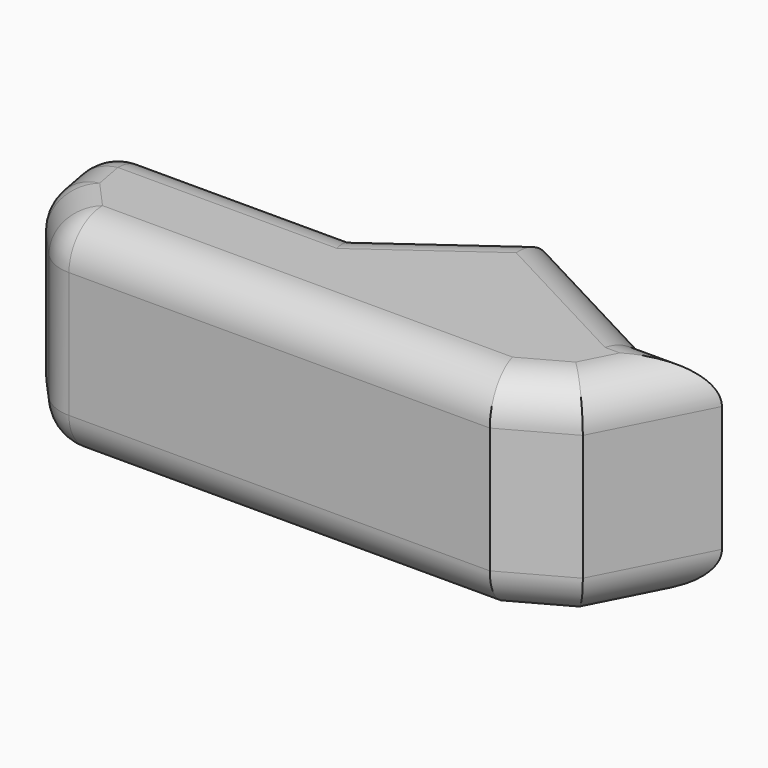
from build123d import *

# Parameters (mm, degrees)
F2_DEPTH     = 25.4
F3_R         = 5.08
F4_T1_DEPTH  = 63.7089962256
F4_T3_DEPTH  = 34.3299805756
F4_T5_DEPTH  = 39.8420593032
F4_T7_DEPTH  = 15.24
F4_T12_DEPTH = 5.08
F4_T18_DEPTH = 5.08
F4_T24_DEPTH = 5.08
F4_T30_DEPTH = 5.08
F4_T36_DEPTH = 37.6403571065
F4_T41_DEPTH = 43.8944483223
F4_T46_DEPTH = 48.4484626095
F4_T51_DEPTH = 34.2442917913
F4_T57_DEPTH = 43.8944483223
F4_T61_DEPTH = 37.6403571065
F4_T68_DEPTH = 48.4484626095
F4_T72_DEPTH = 34.2442917913


# Not quite as in the source:
# - a fillet or chamfer that OpenCascade refuses, or shapes differently, is made with other operations: its cross-section is extruded or revolved along the edge and cut away or added


with BuildPart() as f2:
    # F1 (on face) → F2 (new body)
    with BuildSketch(Plane.XY):
        Polygon((8.4329312667, 10.7982652262), (-6.5817977302, 0), (-37.6396663487, 0), (-35.5828553438, -11.0039459541), (-30.0294607878, -17.1743836254), (23.241976276, -17.1743836254), (31.0578662902, -12.8550762311), (37.6396663487, 0), (28.7953745574, 0), align=None)
    extrude(amount=F2_DEPTH)

    # F3
    f3_edges = [f2.edges().sort_by_distance(p)[0] for p in [
        (-22.110732, 0, 25.4),
        (18.614153, 5.399133, 25.4),
        (33.21752, 0, 25.4),
        (34.348766, -6.427538, 25.4),
        (27.149921, -15.01473, 25.4),
        (-3.393742, -17.174384, 25.4),
        (-32.806158, -14.089165, 25.4),
        (-36.611261, -5.501973, 25.4),
        (-32.806158, -14.089165, 0),
        (-36.611261, -5.501973, 0),
        (-35.582855, -11.003946, 12.7),
        (0.925567, 5.399133, 25.4),
    ]]
    fillet(f3_edges, radius=F3_R)

    # F4: fillet of radius 5.08 on 11 edges, made by hand

    # F4_s2 → F4_t1 (cut)
    with BuildSketch(Plane.YZ.offset(-27.7670199495)):
        with BuildLine():
            ThreePointArc((-12.0943836254, 0), (-15.6864860738, 1.4878975516), (-17.1743836254, 5.08))
            Line((-17.1743836254, 5.08), (-17.1743836254, 0))
            Line((-17.1743836254, 0), (-12.0943836254, 0))
        make_face()
    extrude(amount=F4_T1_DEPTH, mode=Mode.SUBTRACT)

    # F4_s4 → F4_t3 (cut)
    with BuildSketch(Plane(origin=(-0.5817443509, -0.3214902809, 0), x_dir=(0, 0, 1), z_dir=(0.8752415471, 0.4836860907, 0))):
        with BuildLine():
            ThreePointArc((0, 21.1935547384), (1.4878975516, 24.7856571868), (5.08, 26.2735547384))
            Line((5.08, 26.2735547384), (0, 26.2735547384))
            Line((0, 26.2735547384), (0, 21.1935547384))
        make_face()
    extrude(amount=F4_T3_DEPTH, mode=Mode.SUBTRACT)

    # F4_s6 → F4_t5 (cut)
    with BuildSketch(Plane(origin=(-4.5520149502, -8.8906528107, 0), x_dir=(0, 0, 1), z_dir=(0.4557383348, 0.8901137962, 0))):
        with BuildLine():
            ThreePointArc((0, 28.4235863007), (1.4878975516, 32.0156887492), (5.08, 33.5035863007))
            Line((5.08, 33.5035863007), (0, 33.5035863007))
            Line((0, 33.5035863007), (0, 28.4235863007))
        make_face()
    extrude(amount=F4_T5_DEPTH, mode=Mode.SUBTRACT)

    # F4_s8 → F4_t7 (cut)
    with BuildSketch(Plane.XY.offset(5.08)):
        with BuildLine():
            ThreePointArc((-31.5221548367, 0), (-35.430345336, -1.8346268287), (-36.5156731811, -6.0133673145))
            Line((-36.5156731811, -6.0133673145), (-37.6396663487, 0))
            Line((-37.6396663487, 0), (-31.5221548367, 0))
        make_face()
        with BuildLine():
            ThreePointArc((-27.7670199495, -17.1743836254), (-29.8337598255, -16.7349640077), (-31.5429540141, -15.4927246824))
            Line((-31.5429540141, -15.4927246824), (-30.0294607878, -17.1743836254))
            Line((-30.0294607878, -17.1743836254), (-27.7670199495, -17.1743836254))
        make_face()
    extrude(amount=F4_T7_DEPTH, mode=Mode.SUBTRACT)


with BuildPart() as f4_tool10:
    # F4_s11 → F4_t12 (new body)
    with BuildSketch(Plane.XY.offset(20.32)):
        Polygon((-27.7670199495, -12.0943836254), (-27.7670199495, -17.1743836254), (-30.0294607878, -17.1743836254), (-31.5429540141, -15.4927246824), align=None)
    extrude(amount=F4_T12_DEPTH)

    # F4_s13 → F4_t14 (revolve, cut)
    with BuildSketch(Plane(origin=(-27.7670199495, -12.0943836254, 20.32), x_dir=(0.4068385583, 0.9135000753, 0), z_dir=(0.9135000753, -0.4068385583, 0))):
        with BuildLine():
            ThreePointArc((0, -5.08), (5.08, 0), (0, 5.08))
            Line((0, 5.08), (0, -5.08))
        make_face()
    revolve(axis=Axis((-27.7670199495, -12.0943836254, 20.32), (0, 0, 1)), mode=Mode.SUBTRACT)


with BuildPart() as f2_1:
    add(f2.part)

    # F4_t9: cut F4_tool10
    add(f4_tool10.part, mode=Mode.SUBTRACT)


with BuildPart() as f4_tool16:
    # F4_s17 → F4_t18 (new body)
    with BuildSketch(Plane.XY.offset(20.32)):
        Polygon((-31.5221548367, -5.08), (-31.5221548367, 0), (-37.6396663487, 0), (-36.5156731811, -6.0133673145), align=None)
    extrude(amount=F4_T18_DEPTH)

    # F4_s19 → F4_t20 (revolve, cut)
    with BuildSketch(Plane(origin=(-31.5221548367, -5.08, 20.32), x_dir=(0.7693288384, -0.6388529865, 0), z_dir=(-0.6388529865, -0.7693288384, 0))):
        with BuildLine():
            ThreePointArc((0, -5.08), (5.08, 0), (0, 5.08))
            Line((0, 5.08), (0, -5.08))
        make_face()
    revolve(axis=Axis((-31.5221548367, -5.08, 20.32), (0, 0, 1)), mode=Mode.SUBTRACT)


with BuildPart() as f2_2:
    add(f2_1.part)

    # F4_t15: cut F4_tool16
    add(f4_tool16.part, mode=Mode.SUBTRACT)


with BuildPart() as f4_tool22:
    # F4_s23 → F4_t24 (new body)
    with BuildSketch(Plane.XY.offset(5.08)):
        Polygon((-27.7670199495, -12.0943836254), (-27.7670199495, -17.1743836254), (-30.0294607878, -17.1743836254), (-31.5429540141, -15.4927246824), align=None)
    extrude(amount=-F4_T24_DEPTH)

    # F4_s25 → F4_t26 (revolve, cut)
    with BuildSketch(Plane(origin=(-27.7670199495, -12.0943836254, 5.08), x_dir=(0.4068385583, 0.9135000753, 0), z_dir=(-0.9135000753, 0.4068385583, 0))):
        with BuildLine():
            ThreePointArc((0, -5.08), (5.08, 0), (0, 5.08))
            Line((0, 5.08), (0, -5.08))
        make_face()
    revolve(axis=Axis((-27.7670199495, -12.0943836254, 5.08), (0, 0, -1)), mode=Mode.SUBTRACT)


with BuildPart() as f2_3:
    add(f2_2.part)

    # F4_t21: cut F4_tool22
    add(f4_tool22.part, mode=Mode.SUBTRACT)


with BuildPart() as f4_tool28:
    # F4_s29 → F4_t30 (new body)
    with BuildSketch(Plane.XY.offset(5.08)):
        Polygon((-31.5221548367, -5.08), (-31.5221548367, 0), (-37.6396663487, 0), (-36.5156731811, -6.0133673145), align=None)
    extrude(amount=-F4_T30_DEPTH)

    # F4_s31 → F4_t32 (revolve, cut)
    with BuildSketch(Plane(origin=(-31.5221548367, -5.08, 5.08), x_dir=(0.7693288384, -0.6388529865, 0), z_dir=(0.6388529865, 0.7693288384, 0))):
        with BuildLine():
            ThreePointArc((0, -5.08), (5.08, 0), (0, 5.08))
            Line((0, 5.08), (0, -5.08))
        make_face()
    revolve(axis=Axis((-31.5221548367, -5.08, 5.08), (0, 0, -1)), mode=Mode.SUBTRACT)


with BuildPart() as f2_4:
    add(f2_3.part)

    # F4_t27: cut F4_tool28
    add(f4_tool28.part, mode=Mode.SUBTRACT)


with BuildPart() as f4_tool34:
    # F4_s35 → F4_t36 (new body)
    with BuildSketch(Plane.YZ.offset(6.1182022698)):
        with BuildLine():
            ThreePointArc((-5.08, 0), (-1.4878975516, 1.4878975516), (0, 5.08))
            Line((0, 5.08), (0, 0))
            Line((0, 0), (-5.08, 0))
        make_face()
    extrude(amount=-F4_T36_DEPTH)

    split(bisect_by=Plane(origin=(-2.2437256361, 3.119846722, 0), x_dir=(0, 0, 1), z_dir=(-0.5838652247, 0.8118506016, 0)), keep=Keep.TOP)


with BuildPart() as f2_5:
    add(f2_4.part)

    # F4_t33: cut F4_tool34
    add(f4_tool34.part, mode=Mode.SUBTRACT)


with BuildPart() as f4_tool39:
    # F4_s40 → F4_t41 (new body)
    with BuildSketch(Plane(origin=(20.9871595433, 15.0935068584, 0), x_dir=(0, 0, 1), z_dir=(-0.8118506016, -0.5838652247, 0))):
        with BuildLine():
            ThreePointArc((5.08, 3.8428828109), (1.4878975516, 2.3549852594), (0, -1.2371171891))
            Line((0, -1.2371171891), (0, 3.8428828109))
            Line((0, 3.8428828109), (5.08, 3.8428828109))
        make_face()
    extrude(amount=F4_T41_DEPTH)

    split(bisect_by=Plane.XZ, keep=Keep.BOTTOM)


with BuildPart() as f2_6:
    add(f2_5.part)

    # F4_t38: cut F4_tool39
    add(f4_tool39.part, mode=Mode.SUBTRACT)


with BuildPart() as f4_tool44:
    # F4_s45 → F4_t46 (new body)
    with BuildSketch(Plane(origin=(33.6949109219, -17.8685131108, 0), x_dir=(0, 0, 1), z_dir=(-0.8834621049, 0.4685026246, 0))):
        with BuildLine():
            ThreePointArc((5.08, 13.4907085573), (1.4878975516, 12.0028110057), (0, 8.4107085573))
            Line((0, 8.4107085573), (0, 13.4907085573))
            Line((0, 13.4907085573), (5.08, 13.4907085573))
        make_face()
    extrude(amount=F4_T46_DEPTH)

    split(bisect_by=Plane.XZ, keep=Keep.BOTTOM)


with BuildPart() as f2_7:
    add(f2_6.part)

    # F4_t43: cut F4_tool44
    add(f4_tool44.part, mode=Mode.SUBTRACT)


with BuildPart() as f4_tool49:
    # F4_s50 → F4_t51 (new body)
    with BuildSketch(Plane.YZ.offset(50.3396663487)):
        with BuildLine():
            ThreePointArc((-5.08, 0), (-1.4878975516, 1.4878975516), (0, 5.08))
            Line((0, 5.08), (0, 0))
            Line((0, 0), (-5.08, 0))
        make_face()
    extrude(amount=-F4_T51_DEPTH)

    split(bisect_by=Plane(origin=(6.3204323672, 11.918529778, 0), x_dir=(0, 0, 1), z_dir=(0.4685026246, 0.8834621049, 0)), keep=Keep.TOP)


with BuildPart() as f2_8:
    add(f2_7.part)

    # F4_t48: cut F4_tool49
    add(f4_tool49.part, mode=Mode.SUBTRACT)


with BuildPart() as f4_tool55:
    # F4_s56 → F4_t57 (new body)
    with BuildSketch(Plane(origin=(20.9871595433, 15.0935068584, 0), x_dir=(0, 0, 1), z_dir=(-0.8118506016, -0.5838652247, 0))):
        with BuildLine():
            ThreePointArc((5.08, 3.8428828109), (1.4878975516, 2.3549852594), (0, -1.2371171891))
            Line((0, -1.2371171891), (0, 3.8428828109))
            Line((0, 3.8428828109), (5.08, 3.8428828109))
        make_face()
    extrude(amount=F4_T57_DEPTH)

    split(bisect_by=Plane.XZ, keep=Keep.TOP)


with BuildPart() as f4_tool59:
    # F4_s60 → F4_t61 (new body)
    with BuildSketch(Plane.YZ.offset(6.1182022698)):
        with BuildLine():
            ThreePointArc((-5.08, 0), (-1.4878975516, 1.4878975516), (0, 5.08))
            Line((0, 5.08), (0, 0))
            Line((0, 0), (-5.08, 0))
        make_face()
    extrude(amount=-F4_T61_DEPTH)

    split(bisect_by=Plane(origin=(-2.2437256361, 3.119846722, 0), x_dir=(0, 0, 1), z_dir=(0.5838652247, -0.8118506016, 0)), keep=Keep.TOP)


with BuildPart() as f4_tool55_1:
    add(f4_tool55.part)

    # F4_t63: intersect F4_tool59
    add(f4_tool59.part, mode=Mode.INTERSECT)


with BuildPart() as f2_9:
    add(f2_8.part)

    # F4_t53: cut F4_tool55
    add(f4_tool55_1.part, mode=Mode.SUBTRACT)


with BuildPart() as f4_tool66:
    # F4_s67 → F4_t68 (new body)
    with BuildSketch(Plane(origin=(33.6949109219, -17.8685131108, 0), x_dir=(0, 0, 1), z_dir=(-0.8834621049, 0.4685026246, 0))):
        with BuildLine():
            ThreePointArc((5.08, 13.4907085573), (1.4878975516, 12.0028110057), (0, 8.4107085573))
            Line((0, 8.4107085573), (0, 13.4907085573))
            Line((0, 13.4907085573), (5.08, 13.4907085573))
        make_face()
    extrude(amount=F4_T68_DEPTH)

    split(bisect_by=Plane.XZ, keep=Keep.TOP)


with BuildPart() as f4_tool70:
    # F4_s71 → F4_t72 (new body)
    with BuildSketch(Plane.YZ.offset(50.3396663487)):
        with BuildLine():
            ThreePointArc((-5.08, 0), (-1.4878975516, 1.4878975516), (0, 5.08))
            Line((0, 5.08), (0, 0))
            Line((0, 0), (-5.08, 0))
        make_face()
    extrude(amount=-F4_T72_DEPTH)

    split(bisect_by=Plane(origin=(6.3204323672, 11.918529778, 0), x_dir=(0, 0, 1), z_dir=(-0.4685026246, -0.8834621049, 0)), keep=Keep.TOP)


with BuildPart() as f4_tool66_1:
    add(f4_tool66.part)

    # F4_t74: intersect F4_tool70
    add(f4_tool70.part, mode=Mode.INTERSECT)


with BuildPart() as f2_10:
    add(f2_9.part)

    # F4_t64: cut F4_tool66
    add(f4_tool66_1.part, mode=Mode.SUBTRACT)


solid = f2_10.part
